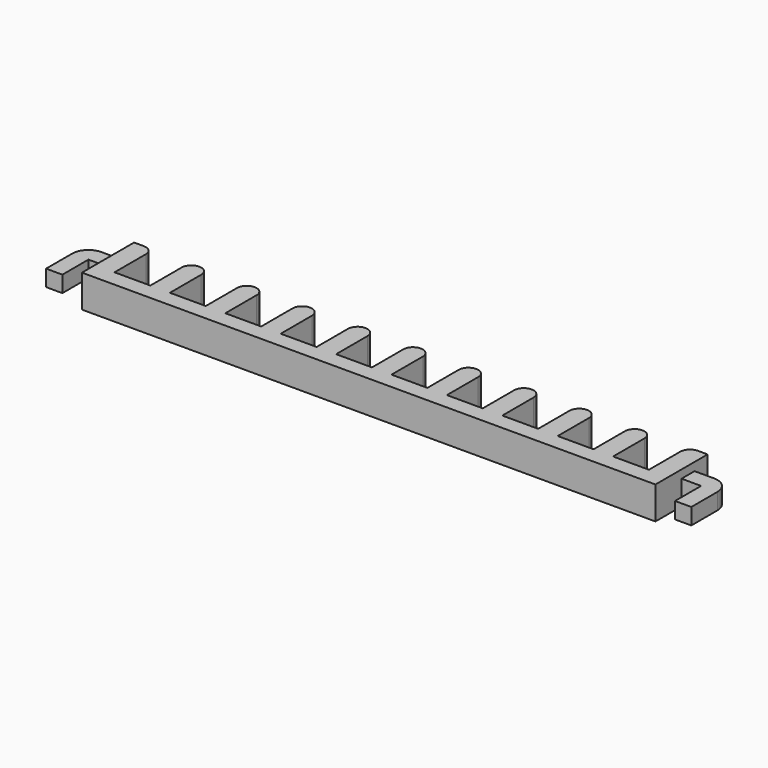
from build123d import *

# Parameters (mm, degrees)
F1_DEPTH  = 10
F2_W      = 5
F2_H      = 5
F3_DEPTH  = 11
F4_W      = 5
F4_H      = 5
F5_DEPTH  = 10
F6_R      = 2.99999
F7_R      = 5
F8_W      = 5
F8_H      = 5
F9_DEPTH  = 11
F10_W     = 5
F10_H     = 5
F11_DEPTH = 10
F12_R     = 5


# Not quite as in the source:
# - a fillet or chamfer is up to 0.001 mm smaller than in the source, because OpenCascade refuses the exact size


with BuildPart() as f1:
    # F0 (on Top) → F1 (new body)
    with BuildSketch(Plane.XY):
        Polygon((83, -5), (83, 15), (77, 15), (77, 0), (66, 0), (66, 15), (60, 15), (60, 0), (49, 0), (49, 15), (43, 15), (43, 0), (32, 0), (32, 15), (26, 15), (26, 0), (15, 0), (15, 15), (9, 15), (9, 0), (-2, 0), (-2, 15), (-8, 15), (-8, 0), (-19, 0), (-19, 15), (-25, 15), (-25, 0), (-36, 0), (-36, 15), (-42, 15), (-42, 0), (-53, 0), (-53, 15), (-59, 15), (-59, 0), (-70, 0), (-70, 15), (-76, 15), (-76, 0), (-87, 0), (-87, 15), (-93, 15), (-93, -5), align=None)
    extrude(amount=F1_DEPTH)

    # F2 (on face) → F3 (join)
    with BuildSketch(Plane(origin=(-93, 0, 0), x_dir=(0, -1, 0), z_dir=(-1, 0, 0))):
        with Locations((-7.5, 5)):
            Rectangle(F2_W, F2_H)
    extrude(amount=F3_DEPTH)

    # F4 (on face) → F5 (join)
    with BuildSketch(Plane.XZ.offset(-5)):
        with Locations((-101.5, 5)):
            Rectangle(F4_W, F4_H)
    extrude(amount=F5_DEPTH)

    # F6 (radius 3 in the source; OpenCascade refuses exactly that, so slightly less here)
    f6_edges = [f1.edges().sort_by_distance(p)[0] for p in [
        (-87, 15, 5),
        (-76, 15, 5),
        (-70, 15, 5),
        (-59, 15, 5),
        (-53, 15, 5),
        (-42, 15, 5),
        (-36, 15, 5),
        (-25, 15, 5),
        (-19, 15, 5),
        (-8, 15, 5),
        (-2, 15, 5),
        (9, 15, 5),
        (15, 15, 5),
        (26, 15, 5),
        (32, 15, 5),
        (43, 15, 5),
        (49, 15, 5),
        (60, 15, 5),
        (66, 15, 5),
        (77, 15, 5),
    ]]
    fillet(f6_edges, radius=F6_R)

    # F7
    f7_edges = [f1.edges().sort_by_distance(p)[0] for p in [
        (-104, 10, 5),
    ]]
    fillet(f7_edges, radius=F7_R)

    # F8 (on face) → F9 (join)
    with BuildSketch(Plane.YZ.offset(83)):
        with Locations((7.5, 5)):
            Rectangle(F8_W, F8_H)
    extrude(amount=F9_DEPTH)

    # F10 (on face) → F11 (join)
    with BuildSketch(Plane.XZ.offset(-5)):
        with Locations((91.5, 5)):
            Rectangle(F10_W, F10_H)
    extrude(amount=F11_DEPTH)

    # F12
    f12_edges = [f1.edges().sort_by_distance(p)[0] for p in [
        (94, 10, 5),
    ]]
    fillet(f12_edges, radius=F12_R)


solid = f1.part
